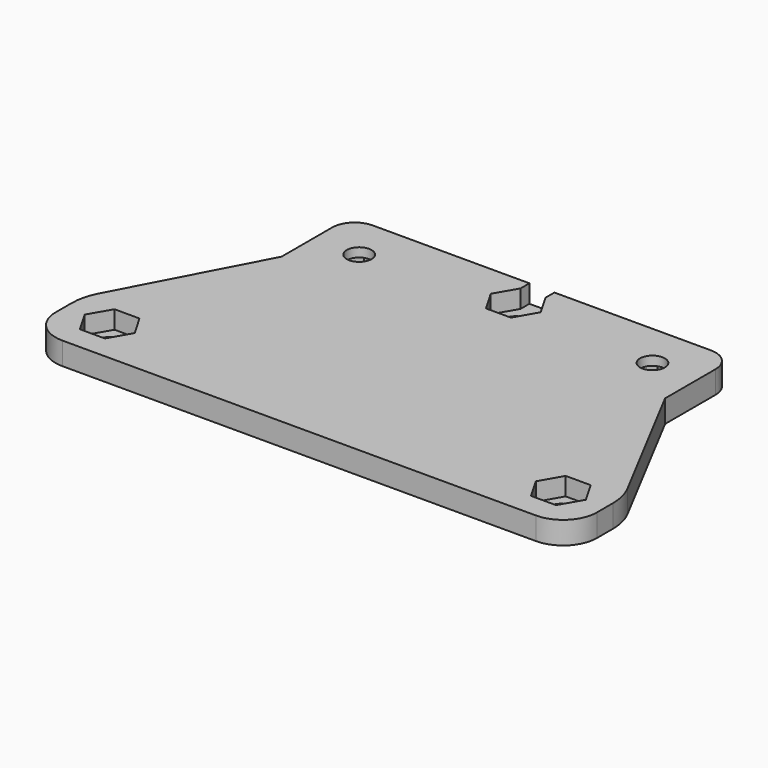
from build123d import *

# Parameters (mm, degrees)
F2_DEPTH = 2
F3_R     = 1.1
F4_DEPTH = 2
F6_DEPTH = 1.2
F7_W     = 2.2170250337
F7_H     = 0.98
F8_DEPTH = 1.6
F9_R     = 2
F10_R    = 5
F11_R    = 3


with BuildPart() as f2:
    # F1 (on Top) → F2 (new body)
    with BuildSketch(Plane.XY):
        Polygon((0, 4), (-3, 4), (-13, 4), (-17, 4), (-17, -3.6), (-24, -16.9), (-24, -22.9), (0, -22.9), (24, -22.9), (24, -16.9), (17, -3.6), (17, 4), (13, 4), (3, 4), align=None)
    extrude(amount=F2_DEPTH)

    # F3 (on face) → F4 (cut, through all)
    with BuildSketch(Plane(origin=(0, 0, 0), x_dir=(1, 0, 0), z_dir=(0, 0, -1))):
        with Locations((20, 18.9)):
            Circle(F3_R)
        with Locations((13, 0)):
            Circle(F3_R)
        with Locations((0, -1.1)):
            Circle(F3_R)
        with Locations((-13, 0)):
            Circle(F3_R)
        with Locations((-20, 18.9)):
            Circle(F3_R)
    extrude(amount=-F4_DEPTH, mode=Mode.SUBTRACT)

    # F5 (on Top) → F6 (cut)
    with BuildSketch(Plane.XY):
        Polygon((10.7829749663, 0), (11.8914874832, -1.92), (14.1085125168, -1.92), (15.2170250337, 0), (14.1085125168, 1.92), (11.8914874832, 1.92), align=None)
        Polygon((-14.1085125168, -1.92), (-11.8914874832, -1.92), (-10.7829749663, 0), (-11.8914874832, 1.92), (-14.1085125168, 1.92), (-15.2170250337, 0), align=None)
    extrude(amount=F6_DEPTH, mode=Mode.SUBTRACT)

    # F7 (on face) → F8 (cut)
    with BuildSketch(Plane.XY.offset(2)):
        Polygon((-17.7829749663, -18.9), (-18.8914874832, -16.98), (-21.1085125168, -16.98), (-22.2170250337, -18.9), (-21.1085125168, -20.82), (-18.8914874832, -20.82), align=None)
        with Locations((0, 3.51)):
            Rectangle(F7_W, F7_H)
        Polygon((1.1085125168, 3.02), (-1.1085125168, 3.02), (-2.2170250337, 1.1), (-1.1085125168, -0.82), (1.1085125168, -0.82), (2.2170250337, 1.1), align=None)
        Polygon((18.8914874832, -16.98), (17.7829749663, -18.9), (18.8914874832, -20.82), (21.1085125168, -20.82), (22.2170250337, -18.9), (21.1085125168, -16.98), align=None)
    extrude(amount=-F8_DEPTH, mode=Mode.SUBTRACT)

    # F9
    f9_edges = [f2.edges().sort_by_distance(p)[0] for p in [
        (-17, 4, 1),
        (17, 4, 1),
    ]]
    fillet(f9_edges, radius=F9_R)

    # F10
    f10_edges = [f2.edges().sort_by_distance(p)[0] for p in [
        (24, -16.9, 1),
        (-24, -16.9, 1),
    ]]
    fillet(f10_edges, radius=F10_R)

    # F11
    f11_edges = [f2.edges().sort_by_distance(p)[0] for p in [
        (24, -22.9, 1),
        (-24, -22.9, 1),
    ]]
    fillet(f11_edges, radius=F11_R)


solid = f2.part
